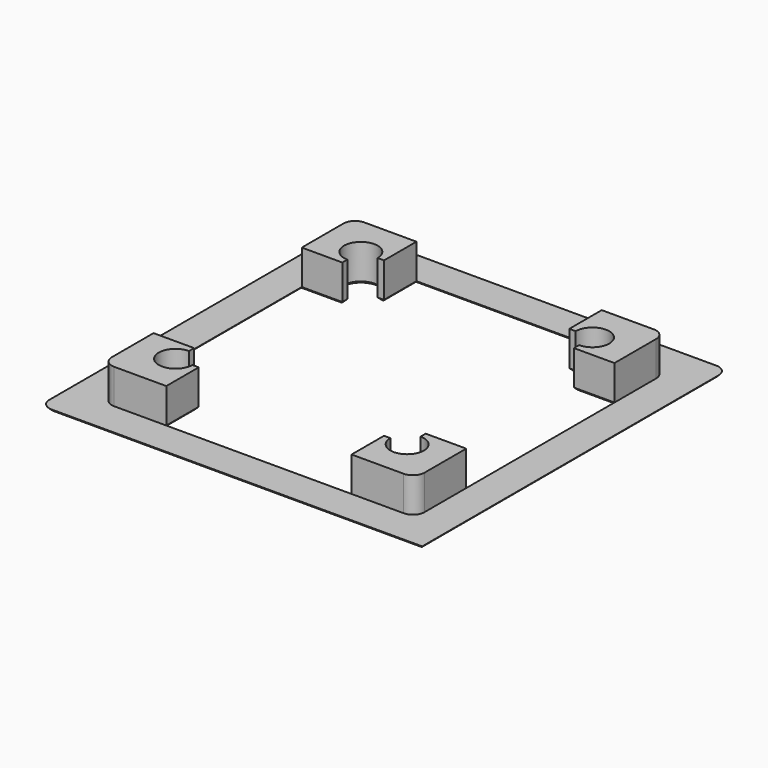
from build123d import *

# Parameters (mm, degrees)
F1_R          = 1.45
F6_DEPTH      = 0.201
F6_DEPTH_BACK = 3.001
F7_R          = 1
F8_SIZE       = 0.19999


# Not quite as in the source:
# - a fillet or chamfer is up to 0.001 mm smaller than in the source, because OpenCascade refuses the exact size


with BuildPart() as f4:
    # F4: sweep along a path in F2
    with BuildLine(Plane.XZ) as f4_path:
        Line((0, 0), (0, -0.2))
    # F3 (on Top) → F4 (sweep)
    with BuildSketch(Plane.XY):
        Polygon((16.5, 16.5), (0, 16.5), (-16.5, 16.5), (-16.5, 0), (-16.5, -16.5), (0, -16.5), (16.5, -16.5), (16.5, 0), align=None)
        Polygon((0, 13.5), (8, 13.5), (13.5, 13.5), (13.5, 8), (13.5, 0), (13.5, -8), (13.5, -13.5), (8, -13.5), (0, -13.5), (-8, -13.5), (-13.5, -13.5), (-13.5, -8), (-13.5, 0), (-13.5, 8), (-13.5, 13.5), (-8, 13.5), align=None, mode=Mode.SUBTRACT)
        Polygon((-10, -8), (-13.5, -8), (-13.5, -13.5), (-8, -13.5), (-8, -10), (-10, -10), align=None)
        Polygon((-8, 10), (-8, 13.5), (-13.5, 13.5), (-13.5, 8), (-10, 8), (-10, 10), align=None)
        Polygon((8, 13.5), (8, 10), (10, 10), (10, 8), (13.5, 8), (13.5, 13.5), align=None)
        Polygon((13.5, -13.5), (13.5, -8), (10, -8), (10, -10), (8, -10), (8, -13.5), align=None)
    sweep(path=f4_path.line)

    # F5: sweep along a path in F2
    with BuildLine(Plane.XZ) as f5_path:
        Line((0, 0), (0, 3))
    # F3 (on Top) → F5 (sweep)
    with BuildSketch(Plane.XY):
        Polygon((-8, 10), (-8, 13.5), (-13.5, 13.5), (-13.5, 8), (-10, 8), (-10, 10), align=None)
        Polygon((8, 13.5), (8, 10), (10, 10), (10, 8), (13.5, 8), (13.5, 13.5), align=None)
        Polygon((-10, -8), (-13.5, -8), (-13.5, -13.5), (-8, -13.5), (-8, -10), (-10, -10), align=None)
        Polygon((13.5, -13.5), (13.5, -8), (10, -8), (10, -10), (8, -10), (8, -13.5), align=None)
    sweep(path=f5_path.line)

    # F1 (on Top) → F6 (cut, two sides)
    with BuildSketch(Plane.XY) as f6_sk:
        with Locations((10, 10)):
            Circle(F1_R)
        with Locations((-10, 10)):
            Circle(F1_R)
        with Locations((-10, -10)):
            Circle(F1_R)
        with Locations((10, -10)):
            Circle(F1_R)
    extrude(amount=-F6_DEPTH, mode=Mode.SUBTRACT)
    extrude(f6_sk.sketch, amount=F6_DEPTH_BACK, mode=Mode.SUBTRACT)

    # F7
    f7_edges = [f4.edges().sort_by_distance(p)[0] for p in [
        (16.5, 16.5, -0.1),
        (13.5, -13.5, 1.5),
        (13.5, 13.5, 1.5),
        (-13.5, -13.5, 1.5),
        (-16.5, -16.5, -0.1),
        (-13.5, 13.5, 1.5),
        (-16.5, 16.5, -0.1),
    ]]
    fillet(f7_edges, radius=F7_R)

    # F8 (size 0.2 in the source; OpenCascade refuses exactly that, so slightly less here)
    f8_edges = [f4.edges().sort_by_distance(p)[0] for p in [
        (0, 16.5, -0.2),
        (16.207107, 16.207107, -0.2),
        (-16.207107, 16.207107, -0.2),
        (16.5, -0.5, -0.2),
        (-16.5, 0, -0.2),
        (0.5, -16.5, -0.2),
        (-16.207107, -16.207107, -0.2),
        (-13.5, 0, -0.2),
        (-11.75, 8, -0.2),
        (-10, 8.275, -0.2),
        (-11.025305, 11.025305, -0.2),
        (-8.275, 10, -0.2),
        (-8, 11.75, -0.2),
        (0, 13.5, -0.2),
        (8, 11.75, -0.2),
        (8.275, 10, -0.2),
        (11.025305, 11.025305, -0.2),
        (10, 8.275, -0.2),
        (11.75, 8, -0.2),
        (13.5, 0, -0.2),
        (11.75, -8, -0.2),
        (10, -8.275, -0.2),
        (11.025305, -11.025305, -0.2),
        (8.275, -10, -0.2),
        (8, -11.75, -0.2),
        (0, -13.5, -0.2),
        (-8, -11.75, -0.2),
        (-8.275, -10, -0.2),
        (-11.025305, -11.025305, -0.2),
        (-10, -8.275, -0.2),
        (-11.75, -8, -0.2),
    ]]
    chamfer(f8_edges, length=F8_SIZE)


solid = f4.part
